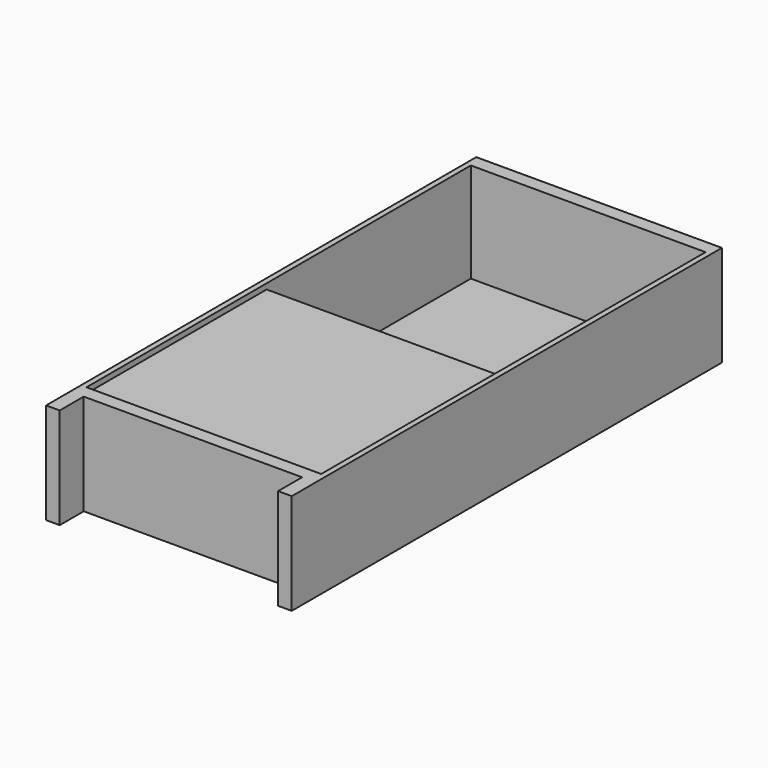
from build123d import *

# Parameters (mm, degrees)
F1_DEPTH = 370
F0_W     = 860
F0_H     = 825
F0_H_2   = 935
F2_DEPTH = 5
F4_DEPTH = 350


with BuildPart() as f1:
    # F0 (on Top) → F1 (new body)
    with BuildSketch(Plane.XY):
        Polygon((450, 985), (-450, 985), (-450, -985), (-400, -985), (-400, -875), (400, -875), (400, -985), (450, -985), align=None)
        Polygon((430, -825), (-430, -825), (-430, 0), (-430, 935), (430, 935), (430, 0), align=None, mode=Mode.SUBTRACT)
    extrude(amount=F1_DEPTH)

    # F0 (on Top) → F2 (join)
    with BuildSketch(Plane.XY):
        with Locations((0, -412.5)):
            Rectangle(F0_W, F0_H)
        with Locations((0, 467.5)):
            Rectangle(F0_W, F0_H_2)
    extrude(amount=F2_DEPTH)


with BuildPart() as f3_1:
    # F3: copy of F1
    add(f1.part)


with BuildPart() as f1_1:
    add(f1.part)

    # F0 (on Top) → F4 (join)
    with BuildSketch(Plane.XY):
        with Locations((0, -412.5)):
            Rectangle(F0_W, F0_H)
    extrude(amount=F4_DEPTH)


solid = Compound([f3_1.part, f1_1.part])
